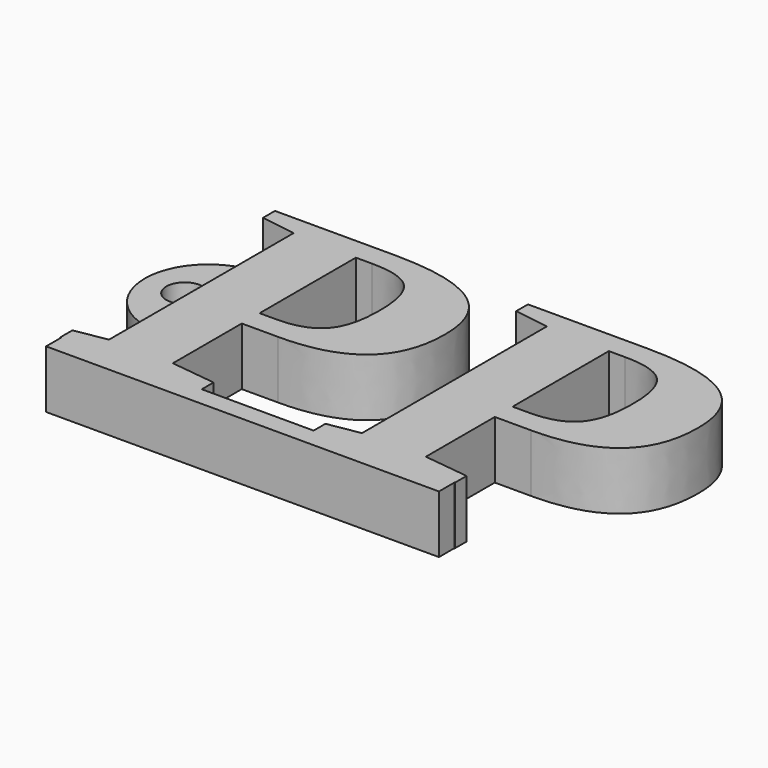
from build123d import *

# Parameters (mm, degrees)
F1_DEPTH = 5
F0_R     = 1.5875
F2_DEPTH = 3.5


# Not quite as in the source:
# - a feature names something its author has since deleted; it is built from what else it names


with BuildPart() as f1:
    # F0 (on Top) → F1 (new body)
    with BuildSketch(Plane.XY):
        with BuildLine():
            Line((-27.2502941939, 1.753040044), (-27.1751960216, 1.753040044))
            Line((-27.1751960216, 1.753040044), (-15.0386480573, 1.753040044))
            Line((-15.0386480573, 1.753040044), (-15.0386480573, 3.0296357887))
            Line((-15.0386480573, 3.0296357887), (-18.9412236452, 3.5055596409))
            Line((-18.9412236452, 3.5055596409), (-18.9412236452, 10.9579672556))
            Line((-18.9412236452, 10.9579672556), (-15.7889280125, 10.9579672556))
            add(Edge.make_bspline(
                [(-7.216699569, 18.3039918917), (-7.216699569, 10.9579672556), (-15.7889280125, 10.9579672556)],
                knots=[0, 0, 0, 1, 1, 1], degree=2))
            add(Edge.make_bspline(
                [(-9.6831049442, 23.5475529219), (-7.216699569, 21.8762203352), (-7.216699569, 18.3039918917)],
                knots=[0, 0, 0, 1, 1, 1], degree=2))
            add(Edge.make_bspline(
                [(-17.138312111, 25.2188855087), (-12.1495103193, 25.2188855087), (-9.6831049442, 23.5475529219)],
                knots=[0, 0, 0, 1, 1, 1], degree=2))
            Line((-17.138312111, 25.2188855087), (-27.4798574638, 25.2188855087))
            Line((-27.4798574638, 25.2188855087), (-27.4798574638, 23.942289764))
            Line((-27.4798574638, 23.942289764), (-24.4675394346, 23.4831632243))
            Line((-24.4675394346, 23.4831632243), (-24.4675394346, 19.757044316))
            ThreePointArc((-24.4675394346, 19.757044316), (-20.580748307, 18.1448768508), (-18.9710911065, 14.2570454627))
            ThreePointArc((-18.9710911065, 14.2570454627), (-20.580748307, 10.3692140746), (-24.4675394346, 8.7570466095))
            Line((-24.4675394346, 8.7570466095), (-24.4675394346, 3.5055596409))
            Line((-24.4675394346, 3.5055596409), (-27.2502941939, 3.0296357887))
            Line((-27.2502941939, 3.0296357887), (-27.2502941939, 1.753040044))
        make_face()
        with BuildLine():
            add(Edge.make_bspline(
                [(-12.8493983372, 18.2703972668), (-12.8493983372, 21.0699493385), (-13.8908317079, 22.181371511)],
                knots=[0, 0, 0, 1, 1, 1], degree=2))
            add(Edge.make_bspline(
                [(-13.9524218535, 14.1074633363), (-12.8493983372, 15.3308675916), (-12.8493983372, 18.2703972668)],
                knots=[0, 0, 0, 1, 1, 1], degree=2))
            add(Edge.make_bspline(
                [(-17.4854565679, 12.884059081), (-15.0554453697, 12.884059081), (-13.9524218535, 14.1074633363)],
                knots=[0, 0, 0, 1, 1, 1], degree=2))
            Line((-17.4854565679, 12.884059081), (-18.9412236452, 12.884059081))
            Line((-18.9412236452, 12.884059081), (-18.9412236452, 23.2927936834))
            Line((-18.9412236452, 23.2927936834), (-17.5582449218, 23.2927936834))
            add(Edge.make_bspline(
                [(-13.8908317079, 22.181371511), (-14.9322650785, 23.2927936834), (-17.5582449218, 23.2927936834)],
                knots=[0, 0, 0, 1, 1, 1], degree=2))
        make_face(mode=Mode.SUBTRACT)
        Polygon((-15.0386480573, 1.753040044), (-27.1751960216, 1.753040044), (-27.1751960216, 0.0879431242), (6.8105147628, 0.0879431242), (6.8105147628, 1.753040044), (-5.3633960976, 1.753040044), align=None)
        with BuildLine():
            Line((-5.3633960976, 3.0296357887), (-5.3633960976, 1.753040044))
            Line((-5.3633960976, 1.753040044), (6.8105147628, 1.753040044))
            Line((6.8105147628, 1.753040044), (6.848250039, 1.753040044))
            Line((6.848250039, 1.753040044), (6.848250039, 3.0296357887))
            Line((6.848250039, 3.0296357887), (2.9456744511, 3.5055596409))
            Line((2.9456744511, 3.5055596409), (2.9456744511, 10.9579672556))
            Line((2.9456744511, 10.9579672556), (6.0979700838, 10.9579672556))
            add(Edge.make_bspline(
                [(14.6701985273, 18.3039918917), (14.6701985273, 10.9579672556), (6.0979700838, 10.9579672556)],
                knots=[0, 0, 0, 1, 1, 1], degree=2))
            add(Edge.make_bspline(
                [(12.2037931521, 23.5475529219), (14.6701985273, 21.8762203352), (14.6701985273, 18.3039918917)],
                knots=[0, 0, 0, 1, 1, 1], degree=2))
            add(Edge.make_bspline(
                [(4.7485859853, 25.2188855087), (9.737387777, 25.2188855087), (12.2037931521, 23.5475529219)],
                knots=[0, 0, 0, 1, 1, 1], degree=2))
            Line((4.7485859853, 25.2188855087), (-5.5929593675, 25.2188855087))
            Line((-5.5929593675, 25.2188855087), (-5.5929593675, 23.942289764))
            Line((-5.5929593675, 23.942289764), (-2.5806413383, 23.4831632243))
            Line((-2.5806413383, 23.4831632243), (-2.5806413383, 3.5055596409))
            Line((-2.5806413383, 3.5055596409), (-5.3633960976, 3.0296357887))
        make_face()
        with BuildLine():
            add(Edge.make_bspline(
                [(9.0374997591, 18.2703972668), (9.0374997591, 21.0699493385), (7.9960663884, 22.181371511)],
                knots=[0, 0, 0, 1, 1, 1], degree=2))
            add(Edge.make_bspline(
                [(7.9344762428, 14.1074633363), (9.0374997591, 15.3308675916), (9.0374997591, 18.2703972668)],
                knots=[0, 0, 0, 1, 1, 1], degree=2))
            add(Edge.make_bspline(
                [(4.4014415284, 12.884059081), (6.8314527266, 12.884059081), (7.9344762428, 14.1074633363)],
                knots=[0, 0, 0, 1, 1, 1], degree=2))
            Line((4.4014415284, 12.884059081), (2.9456744511, 12.884059081))
            Line((2.9456744511, 12.884059081), (2.9456744511, 23.2927936834))
            Line((2.9456744511, 23.2927936834), (4.3286531745, 23.2927936834))
            add(Edge.make_bspline(
                [(7.9960663884, 22.181371511), (6.9546330178, 23.2927936834), (4.3286531745, 23.2927936834)],
                knots=[0, 0, 0, 1, 1, 1], degree=2))
        make_face(mode=Mode.SUBTRACT)
        with BuildLine():
            Line((-24.4675394346, 19.757044316), (-24.4675394346, 8.7570466095))
            ThreePointArc((-24.4675394346, 8.7570466095), (-20.580748307, 10.3692140746), (-18.9710911065, 14.2570454627))
            ThreePointArc((-18.9710911065, 14.2570454627), (-20.580748307, 18.1448768508), (-24.4675394346, 19.757044316))
        make_face()
    extrude(amount=F1_DEPTH)

    # F0 (on Top) → F2 (join)
    with BuildSketch(Plane.XY):
        with BuildLine():
            ThreePointArc((-24.4675394346, 19.757044316), (-29.9710911065, 14.2570454627), (-24.4675394346, 8.7570466095))
            Line((-24.4675394346, 8.7570466095), (-24.4675394346, 19.757044316))
        make_face()
        with Locations((-26.5210345387, 14.2570454627)):
            Circle(F0_R, mode=Mode.SUBTRACT)
    extrude(amount=F2_DEPTH)


solid = f1.part
